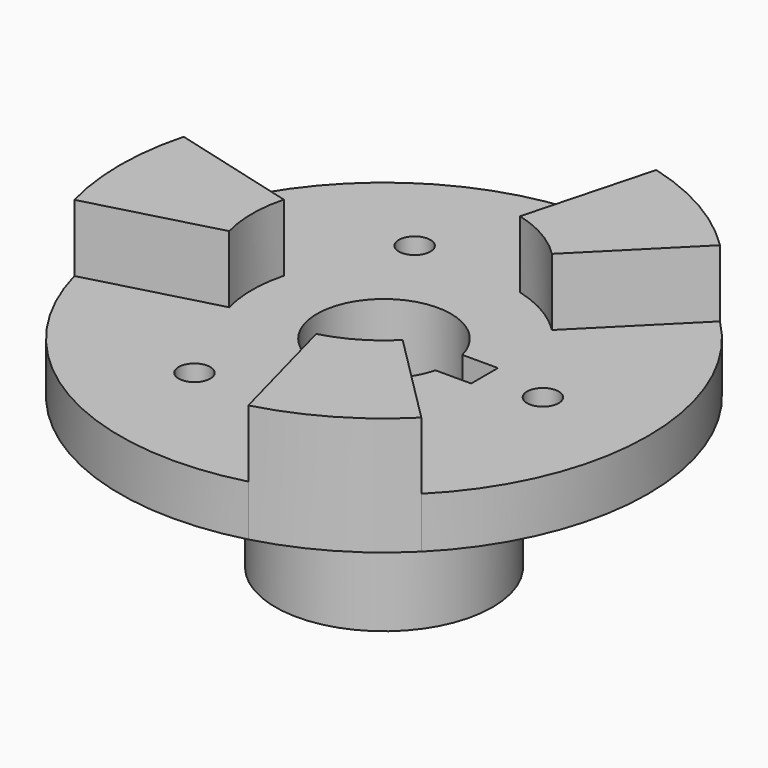
from build123d import *

# Parameters (mm, degrees)
F1_DEPTH = 12.7
F0_R     = 2.9972
F0_R_2   = 20.574
F2_DEPTH = 9.652
F3_DEPTH = 9.652
F4_DEPTH = 38.1


with BuildPart() as f1:
    # F0 (on Top) → F1 (new body)
    with BuildSketch(Plane.XY):
        with BuildLine():
            Line((-24.1480973609, 6.4704631866), (-48.2961947219, 12.9409263732))
            ThreePointArc((-48.2961947219, 12.9409263732), (-49.9999, 0), (-48.2961947219, -12.9409263732))
            Line((-48.2961947219, -12.9409263732), (-24.1480973609, -6.4704631866))
            ThreePointArc((-24.1480973609, -6.4704631866), (-24.99995, 0), (-24.1480973609, 6.4704631866))
        make_face()
    extrude(amount=F1_DEPTH)



with BuildPart() as f1b:
    # F0 (on Top) → F1, piece 2 (new body)
    with BuildSketch(Plane.XY):
        with BuildLine():
            Line((17.6776341743, 17.6776341743), (35.3552683486, 35.3552683486))
            ThreePointArc((35.3552683486, 35.3552683486), (24.99995, 43.3011835867), (12.9409263732, 48.2961947219))
            Line((12.9409263732, 48.2961947219), (6.4704631866, 24.1480973609))
            ThreePointArc((6.4704631866, 24.1480973609), (12.499975, 21.6505917933), (17.6776341743, 17.6776341743))
        make_face()
    extrude(amount=F1_DEPTH)


with BuildPart() as f1c:
    # F0 (on Top) → F1, piece 3 (new body)
    with BuildSketch(Plane.XY):
        with BuildLine():
            ThreePointArc((12.9409263732, -48.2961947219), (24.99995, -43.3011835867), (35.3552683486, -35.3552683486))
            Line((35.3552683486, -35.3552683486), (17.6776341743, -17.6776341743))
            ThreePointArc((17.6776341743, -17.6776341743), (12.499975, -21.6505917933), (6.4704631866, -24.1480973609))
            Line((6.4704631866, -24.1480973609), (12.9409263732, -48.2961947219))
        make_face()
    extrude(amount=F1_DEPTH)


with BuildPart() as f1_1:
    add(f1.part)

    add(f1b.part)  # F2 merges F1b

    add(f1c.part)  # F2 merges F1c
    # F0 (on Top) → F2 (join)
    with BuildSketch(Plane.XY):
        with BuildLine():
            ThreePointArc((35.3552683486, -35.3552683486), (46.1938842376, -19.1341333499), (49.9999, 0))
            ThreePointArc((49.9999, 0), (46.1938842376, 19.1341333499), (35.3552683486, 35.3552683486))
            Line((35.3552683486, 35.3552683486), (17.6776341743, 17.6776341743))
            ThreePointArc((17.6776341743, 17.6776341743), (12.499975, 21.6505917933), (6.4704631866, 24.1480973609))
            Line((6.4704631866, 24.1480973609), (12.9409263732, 48.2961947219))
            ThreePointArc((12.9409263732, 48.2961947219), (-24.99995, 43.3011835867), (-48.2961947219, 12.9409263732))
            Line((-48.2961947219, 12.9409263732), (-24.1480973609, 6.4704631866))
            ThreePointArc((-24.1480973609, 6.4704631866), (-24.99995, 0), (-24.1480973609, -6.4704631866))
            Line((-24.1480973609, -6.4704631866), (-48.2961947219, -12.9409263732))
            ThreePointArc((-48.2961947219, -12.9409263732), (-24.99995, -43.3011835867), (12.9409263732, -48.2961947219))
            Line((12.9409263732, -48.2961947219), (6.4704631866, -24.1480973609))
            ThreePointArc((6.4704631866, -24.1480973609), (12.499975, -21.6505917933), (17.6776341743, -17.6776341743))
            Line((17.6776341743, -17.6776341743), (35.3552683486, -35.3552683486))
        make_face()
        with Locations((-15.0495, -26.0664986285)):
            Circle(F0_R, mode=Mode.SUBTRACT)
        with Locations((-15.0495, 26.0664986285)):
            Circle(F0_R, mode=Mode.SUBTRACT)
        Circle(F0_R_2, mode=Mode.SUBTRACT)
        with Locations((30.099, 0)):
            Circle(F0_R, mode=Mode.SUBTRACT)
        Circle(F0_R_2)
        with BuildLine():
            ThreePointArc((12.2967221242, -3.175), (-12.7, 0), (12.2967221242, 3.175))
            Line((12.2967221242, 3.175), (19.05, 3.175))
            Line((19.05, 3.175), (19.05, 0))
            Line((19.05, 0), (19.05, -3.175))
            Line((19.05, -3.175), (12.2967221242, -3.175))
        make_face(mode=Mode.SUBTRACT)
    extrude(amount=-F2_DEPTH)

    # F3 (add): faces of the model
    f3_faces = [f1_1.faces().sort_by_distance(p)[0] for p in [
        (-38.4460981424, 0, 0),
        (19.2230490712, 33.2952976677, 0),
        (19.2230490712, -33.2952976677, 0),
    ]]
    extrude(f3_faces, amount=F3_DEPTH)

    # F0 (on Top) → F4 (join)
    with BuildSketch(Plane.XY):
        Circle(F0_R_2)
        with BuildLine():
            ThreePointArc((12.2967221242, -3.175), (-12.7, 0), (12.2967221242, 3.175))
            Line((12.2967221242, 3.175), (19.05, 3.175))
            Line((19.05, 3.175), (19.05, 0))
            Line((19.05, 0), (19.05, -3.175))
            Line((19.05, -3.175), (12.2967221242, -3.175))
        make_face(mode=Mode.SUBTRACT)
    extrude(amount=-F4_DEPTH)


solid = f1_1.part
